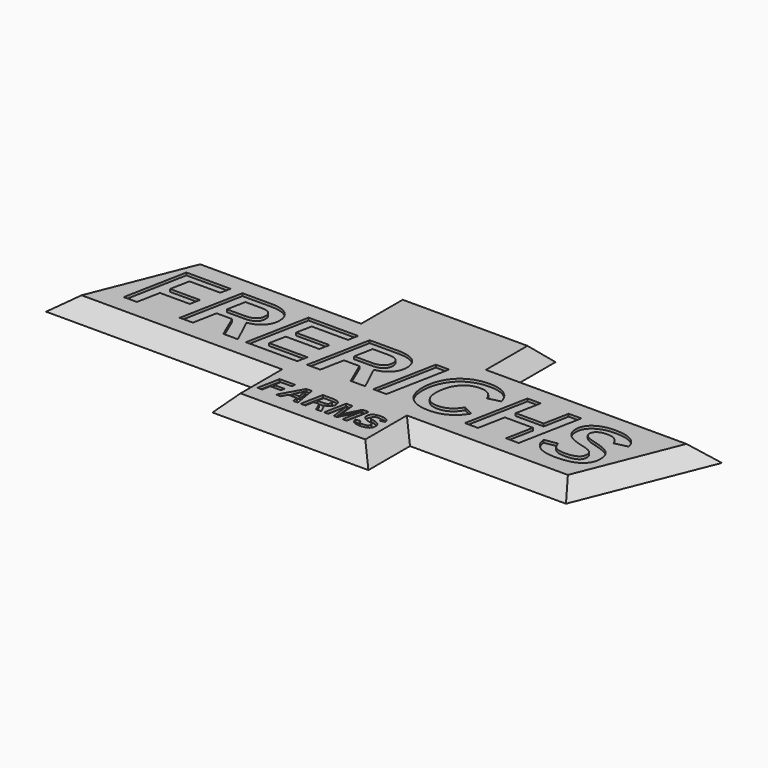
from build123d import *

# Parameters (mm, degrees)
F1_DEPTH       = 7.62
F2_SIZE        = 7.61999
F3_TEXT_SIZE   = 44.7715727259
F3_TEXT_SIZE_2 = 15.812545934
F4_DEPTH       = 1.27


# Not quite as in the source:
# - a fillet or chamfer is up to 0.001 mm smaller than in the source, because OpenCascade refuses the exact size
# - Text() gives the source's letters only with a copy of the font that has no kerning and outlines rounded to 1/6400 em; it was checked with that copy


with BuildPart() as f1:
    # F0 (on Top) → F1 (new body)
    with BuildSketch(Plane.XY):
        Polygon((-114.3, 31.75), (-139.7, -31.75), (-38.1, -31.75), (-38.1, -57.15), (38.1, -57.15), (38.1, -31.75), (114.3, -31.75), (139.7, 31.75), (38.1, 31.75), (38.1, 57.15), (-38.1, 57.15), (-38.1, 31.75), align=None)
    extrude(amount=F1_DEPTH)

    # F2 (size 7.62 in the source; OpenCascade refuses exactly that, so slightly less here)
    f2_edges = [f1.edges().sort_by_distance(p)[0] for p in [
        (-76.2, 31.75, 7.62),
        (-127, 0, 7.62),
        (-88.9, -31.75, 7.62),
        (-38.1, -44.45, 7.62),
        (0, -57.15, 7.62),
        (38.1, -44.45, 7.62),
        (76.2, -31.75, 7.62),
        (127, 0, 7.62),
        (88.9, 31.75, 7.62),
        (38.1, 44.45, 7.62),
        (0, 57.15, 7.62),
        (-38.1, 44.45, 7.62),
    ]]
    chamfer(f2_edges, length=F2_SIZE)

    # F3 (on face) → F4 (cut)
    with BuildSketch(Plane.XY.offset(7.62)):
        with Locations((-115.7450088339, -15.24)):
            Text('FRERICHS', F3_TEXT_SIZE, font='Arimo', font_style=FontStyle.BOLDITALIC, text_align=(TextAlign.LEFT, TextAlign.BOTTOM))
        with Locations((-28.575, -41.8650330725)):
            Text('FARMS', F3_TEXT_SIZE_2, font='Arimo', font_style=FontStyle.BOLDITALIC, text_align=(TextAlign.LEFT, TextAlign.BOTTOM))
    extrude(amount=-F4_DEPTH, mode=Mode.SUBTRACT)


solid = f1.part
